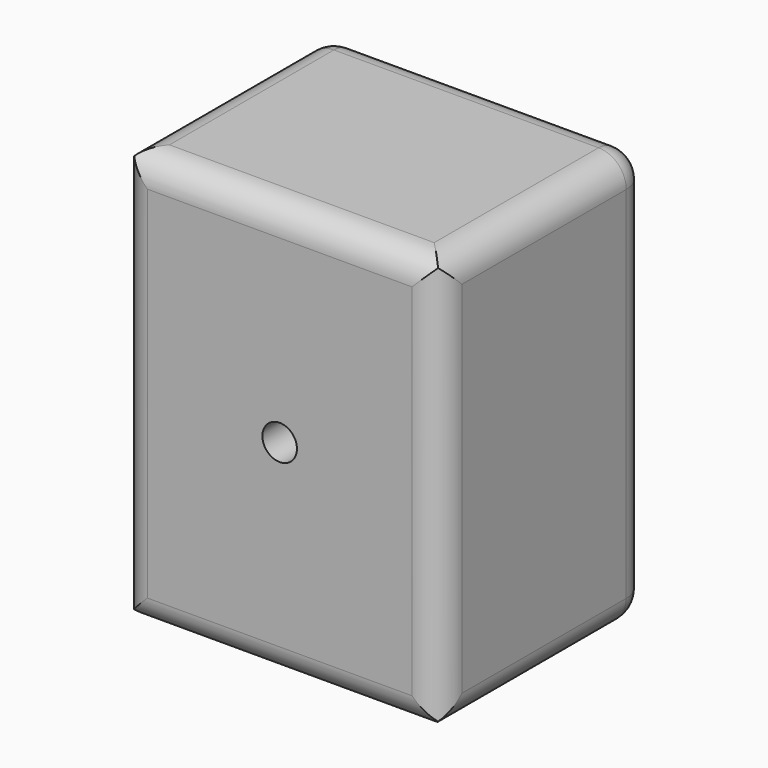
from build123d import *

# Parameters (mm, degrees)
F0_W        = 58.722935617
F0_H        = 47.8591956198
F1_DEPTH    = 76.2
F2_R        = 5.08
F3_T1_DEPTH = 73.962935617
F5_D        = 6.35


# Not quite as in the source:
# - a fillet or chamfer that OpenCascade refuses, or shapes differently, is made with other operations: its cross-section is extruded or revolved along the edge and cut away or added


with BuildPart() as f1:
    # F0 (on Top) → F1 (new body)
    with BuildSketch(Plane.XY):
        Rectangle(F0_W, F0_H)
    extrude(amount=F1_DEPTH)

    # F2
    f2_edges = [f1.edges().sort_by_distance(p)[0] for p in [
        (29.361468, 23.929598, 38.1),
        (0, 23.929598, 76.2),
        (-29.361468, 23.929598, 38.1),
        (0, 23.929598, 0),
        (29.361468, 0, 76.2),
        (29.361468, -23.929598, 38.1),
        (29.361468, 0, 0),
        (-29.361468, 0, 76.2),
        (-29.361468, -23.929598, 38.1),
        (-29.361468, 0, 0),
    ]]
    fillet(f2_edges, radius=F2_R)

    # F3: fillet of radius 5.08 on 4 edges, made by hand

    # F3_s2 → F3_t1 (cut)
    with BuildSketch(Plane.YZ.offset(-36.9814678085)):
        with BuildLine():
            ThreePointArc((-18.8495978099, 0), (-22.4417002583, 1.4878975516), (-23.9295978099, 5.08))
            Line((-23.9295978099, 5.08), (-23.9295978099, 0))
            Line((-23.9295978099, 0), (-18.8495978099, 0))
        make_face()
        with BuildLine():
            ThreePointArc((-18.8495978099, 76.2), (-22.4417002583, 74.7121024484), (-23.9295978099, 71.12))
            Line((-23.9295978099, 71.12), (-23.9295978099, 76.2))
            Line((-23.9295978099, 76.2), (-18.8495978099, 76.2))
        make_face()
    extrude(amount=F3_T1_DEPTH, mode=Mode.SUBTRACT)

    # F5 (through all)
    with Locations(Plane.XZ.offset(23.9295978099)):
        with Locations((0, 38.1)):
            Hole(F5_D / 2)


solid = f1.part
